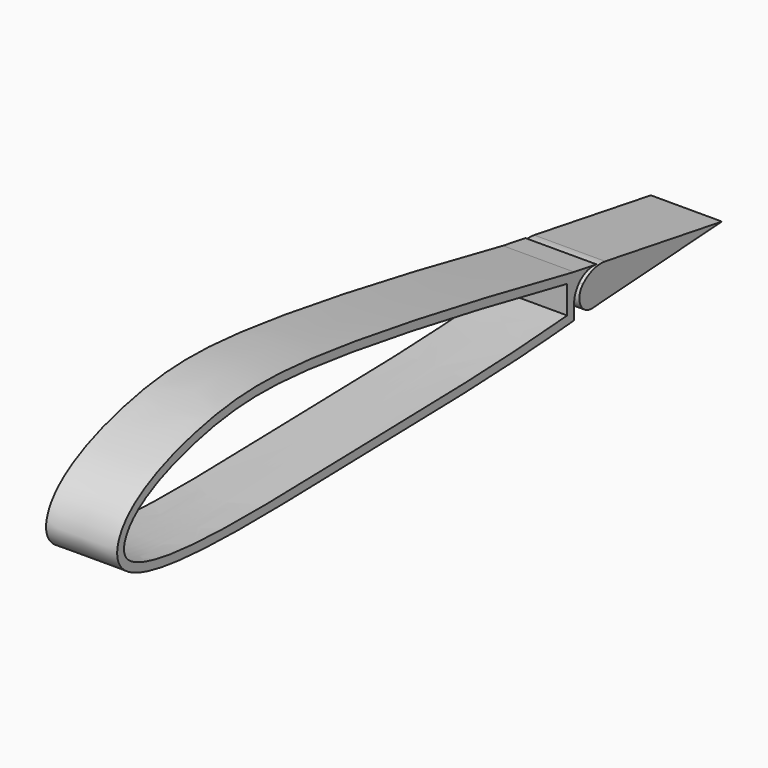
from build123d import *

# Parameters (mm, degrees)
F1_DEPTH  = 25
F4_DEPTH  = 25
F6_DEPTH  = 25
F8_START  = -3
F7_R      = 1.5
F8_DEPTH  = 3
F9_R      = 1.5
F10_DEPTH = 3


# Not quite as in the source:
# - ends of sketch curves that miss each other by under 0.0002 mm in the source are joined
# - the dataset's text gives a spline's control points without its knots; the knots are read off the source's solid


with BuildPart() as f1:
    # F0 (on Right) → F1 (new body)
    with BuildSketch(Plane.YZ):
        with BuildLine():
            add(Edge.make_bspline(
                [(0, 15), (-38.2511828397, 22.9944328087), (-113.6527169167, 37.3957814267), (-159.5763058758, 36.8434374193), (-199.5936407887, 22.7784870475), (-205.2261703216, -7.7748531078), (-89.8624302378, -3.1185538528), (-37.0511047571, -3.2789387286), (0, 0)],
                knots=[0, 0, 0, 0, 0.2265890537, 0.371770979, 0.5009822, 0.5820520045, 0.7880680568, 1, 1, 1, 1], degree=3))
            Line((0, 0), (0, 15))
        make_face()
        with BuildLine():
            Line((-3, 12.5610960382), (-3, 2.7507244211))
            add(Edge.make_bspline(
                [(-3, 12.5610960382), (-7.5138004126, 13.5003832137), (-17.5553922337, 15.5645436399), (-33.4767297194, 18.7358110112), (-50.3871464654, 21.9652165954), (-67.0821604448, 24.9863556376), (-83.1962098823, 27.7000657459), (-95.8344489174, 29.6226188737), (-105.2855428805, 30.9077546106), (-110.8784531171, 31.5952762023), (-115.1406525483, 32.069739408), (-119.2529324322, 32.4917585623), (-124.1294999363, 32.9194147733), (-129.6178799661, 33.2684603631), (-136.5300447572, 33.5095146821), (-142.9538890981, 33.4064583919), (-149.1396038328, 32.9426010414), (-153.7241886486, 32.4091306349), (-157.5531122705, 31.8049649179), (-160.6522106583, 31.2226138954), (-163.7891148662, 30.5728101174), (-167.7654388627, 29.6352846685), (-172.5180409203, 28.3087229623), (-177.1507197739, 26.7807828663), (-181.5595897803, 25.0538522402), (-185.6397785244, 23.1340534366), (-189.2852181566, 21.0337577671), (-191.8725504721, 19.1523135086), (-193.6243664659, 17.587202485), (-194.7685433687, 16.3912035892), (-195.7399405959, 15.1739044697), (-196.8026444586, 13.537578435), (-197.4919221762, 11.9379358185), (-197.8066685808, 10.4707715441), (-197.8666319781, 9.451589737), (-197.7629332855, 8.513723914), (-197.5005435766, 7.6371583365), (-197.0625650465, 6.7893121936), (-196.4057762189, 5.9432145542), (-195.4770067296, 5.0988819558), (-194.1903892216, 4.2381875217), (-192.5617212291, 3.4028712278), (-189.959201776, 2.3513858876), (-185.9598682278, 1.1904625984), (-180.1488723605, 0.0781615219), (-173.485286717, -0.7630128409), (-166.1131330701, -1.3563193981), (-155.5192208175, -1.8564287117), (-144.040599138, -1.9839887458), (-132.1836999682, -1.8734306852), (-123.2258698955, -1.7057942589), (-114.3264252781, -1.4877961992), (-107.0611993818, -1.2928234189), (-101.4001055999, -1.1463048785), (-95.8612110151, -1.0112876887), (-89.1507329437, -0.8599997443), (-81.3878587445, -0.6960715138), (-71.3551119625, -0.4867850333), (-59.2813343866, -0.2161676865), (-45.1265968982, 0.2074746786), (-30.8889867585, 0.8143179941), (-16.9780120063, 1.6395861932), (-7.4648942101, 2.3702924305), (-3, 2.7507244211)],
                knots=[0.0046976742, 0.0046976742, 0.0046976742, 0.0046976742, 0.03125, 0.0625, 0.09375, 0.125, 0.15625, 0.1875, 0.203125, 0.21875, 0.2265625, 0.234375, 0.25, 0.265625, 0.28125, 0.3125, 0.328125, 0.34375, 0.359375, 0.3671875, 0.375, 0.390625, 0.40625, 0.421875, 0.4375, 0.453125, 0.46875, 0.484375, 0.4921875, 0.5, 0.5078125, 0.515625, 0.53125, 0.5390625, 0.546875, 0.5546875, 0.5625, 0.5703125, 0.578125, 0.5859375, 0.59375, 0.6015625, 0.609375, 0.625, 0.640625, 0.65625, 0.671875, 0.6875, 0.71875, 0.734375, 0.75, 0.765625, 0.78125, 0.7890625, 0.796875, 0.8125, 0.828125, 0.84375, 0.875, 0.90625, 0.9375, 0.96875, 0.9947299198, 0.9947299198, 0.9947299198, 0.9947299198], degree=3))
        make_face(mode=Mode.SUBTRACT)
    extrude(amount=F1_DEPTH)

    # F3 (on face) → F4 (join)
    with BuildSketch(Plane(origin=(0, 0, 0), x_dir=(0, -1, 0), z_dir=(-1, 0, 0))):
        with BuildLine():
            ThreePointArc((-9.8644999067, 13.3593776819), (-2.9955873573, 11.4650513076), (0, 5))
            Line((0, 5), (0, 15))
            Line((0, 15), (-9.8644999067, 13.3593776819))
        make_face()
    extrude(amount=-F4_DEPTH)

    # F9 (on face) → F10 (join)
    with BuildSketch(Plane(origin=(0, 0, 0), x_dir=(0, -1, 0), z_dir=(-1, 0, 0))):
        with BuildLine():
            ThreePointArc((-2.4209483757, -9.3970438582), (0.3143477857, -7.5405913323), (2.5, -10.0207496881))
            ThreePointArc((2.5, -10.0207496881), (2.215238736, -11.1795064972), (1.4258261258, -12.0742880634))
            Line((1.4258261258, -12.0742880634), (16.9114564444, -1.3222044655))
            add(Edge.make_bspline(
                [(16.9114564444, -1.3222044655), (11.4748024859, -0.9540485583), (5.8661414584, -0.519140213), (0, 0)],
                knots=[0.9664457304, 0.9664457304, 0.9664457304, 0.9664457304, 1, 1, 1, 1], degree=3))
            Line((0, 0), (-2.4209483757, -9.3970438582))
        make_face()
        with BuildLine():
            ThreePointArc((1.4258261258, -12.0742880634), (2.215238736, -11.1795064972), (2.5, -10.0207496881))
            ThreePointArc((2.5, -10.0207496881), (0.3143477857, -7.5405913323), (-2.4209483757, -9.3970438582))
            ThreePointArc((-2.4209483757, -9.3970438582), (-1.4281023096, -12.0727057776), (1.4258261258, -12.0742880634))
        make_face()
        with Locations((0, -10.0207496881)):
            Circle(F9_R, mode=Mode.SUBTRACT)
    extrude(amount=-F10_DEPTH)


with BuildPart() as f6:
    # F5 (on face) → F6 (new body)
    with BuildSketch(Plane.YZ):
        with BuildLine():
            Line((65, 4.1894721799), (13.7046004851, 12.7207082337))
            ThreePointArc((13.7046004851, 12.7207082337), (8.4507428255, 12.3530611646), (3.9312864889, 9.6488608953))
            ThreePointArc((3.9312864889, 9.6488608953), (10.9962104789, 10.9907828669), (14.9742032146, 5))
            ThreePointArc((14.9742032146, 5), (14.5927644333, 2.8060974013), (13.4932159491, 0.8696838898))
            Line((13.4932159491, 0.8696838898), (65, 4.1894721799))
        make_face()
        with BuildLine():
            ThreePointArc((14.9742032146, 5), (10.9962104789, 10.9907828669), (3.9312864889, 9.6488608953))
            ThreePointArc((3.9312864889, 9.6488608953), (2.7875265162, 3.6662902535), (8.0002776479, 0.5156452406))
            Line((8.0002776479, 0.5156452406), (13.4932159491, 0.8696838898))
            ThreePointArc((13.4932159491, 0.8696838898), (14.5927644333, 2.8060974013), (14.9742032146, 5))
        make_face()
    extrude(amount=F6_DEPTH)

    # F7 (on face) → F8 (join)
    with BuildSketch(Plane(origin=(0, 0, 0), x_dir=(0, -1, 0), z_dir=(-1, 0, 0)).offset(F8_START)):
        with BuildLine():
            Line((-8.0002776479, 0.5156452406), (-23.0002776479, 1.4824465128))
            Line((-23.0002776479, 1.4824465128), (-1.3303406277, -12.1373965207))
            ThreePointArc((-1.3303406277, -12.1373965207), (-1.9959614602, -8.5153800161), (1.6695118525, -8.1599084336))
            Line((1.6695118525, -8.1599084336), (-8.0002776479, 0.5156452406))
        make_face()
        with BuildLine():
            ThreePointArc((1.6695118525, -8.1599084336), (-1.9959614602, -8.5153800161), (-1.3303406277, -12.1373965207))
            ThreePointArc((-1.3303406277, -12.1373965207), (1.2091626091, -12.208882633), (2.5, -10.0207496881))
            ThreePointArc((2.5, -10.0207496881), (2.2829563762, -9.001872765), (1.6695118525, -8.1599084336))
        make_face()
        with Locations((0, -10.0207496881)):
            Circle(F7_R, mode=Mode.SUBTRACT)
    extrude(amount=-F8_DEPTH)


solid = Compound([f1.part, f6.part])
